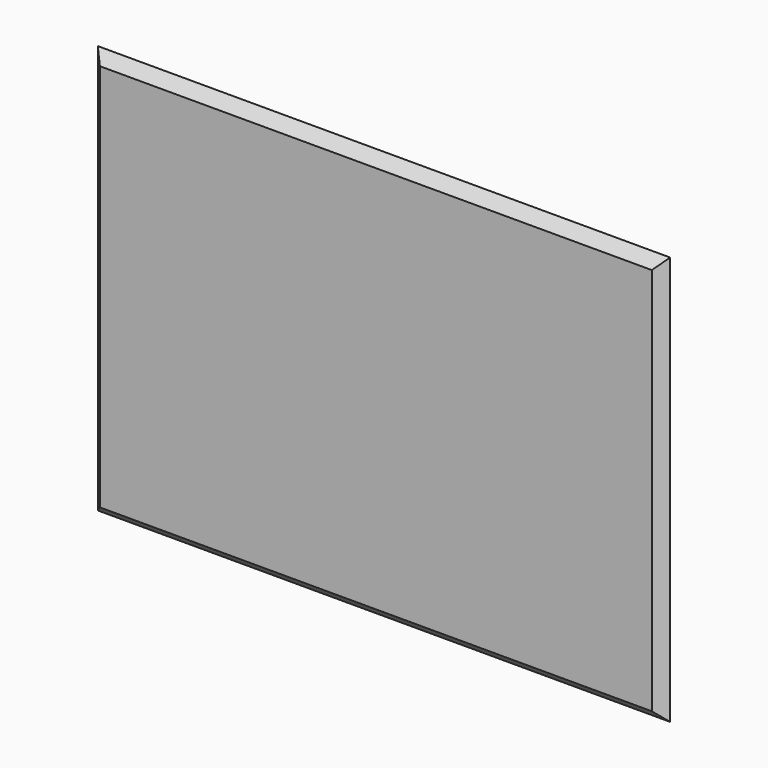
from build123d import *

# Parameters (mm, degrees)
F0_W     = 355.6
F0_H     = 254
F1_DEPTH = 6.35
F2_SIZE2 = 6.34999
F2_SIZE  = 6.34999


# Not quite as in the source:
# - a fillet or chamfer is up to 0.001 mm smaller than in the source, because OpenCascade refuses the exact size


with BuildPart() as f1:
    # F0 (on Front) → F1 (new body)
    with BuildSketch(Plane.XZ):
        with Locations((-3.309763968, 6.3614202906)):
            Rectangle(F0_W, F0_H)
    extrude(amount=F1_DEPTH)

    # F2 (size 6.35 and 6.35 in the source; OpenCascade refuses exactly that, so slightly less here)
    f2_edges = [f1.edges().sort_by_distance(p)[0] for p in [
        (-3.309764, -6.35, 133.36142),
        (-181.109764, -6.35, 6.36142),
        (-3.309764, -6.35, -120.63858),
        (174.490236, -6.35, 6.36142),
    ]]
    chamfer(f2_edges, length=F2_SIZE, length2=F2_SIZE2)


solid = f1.part
